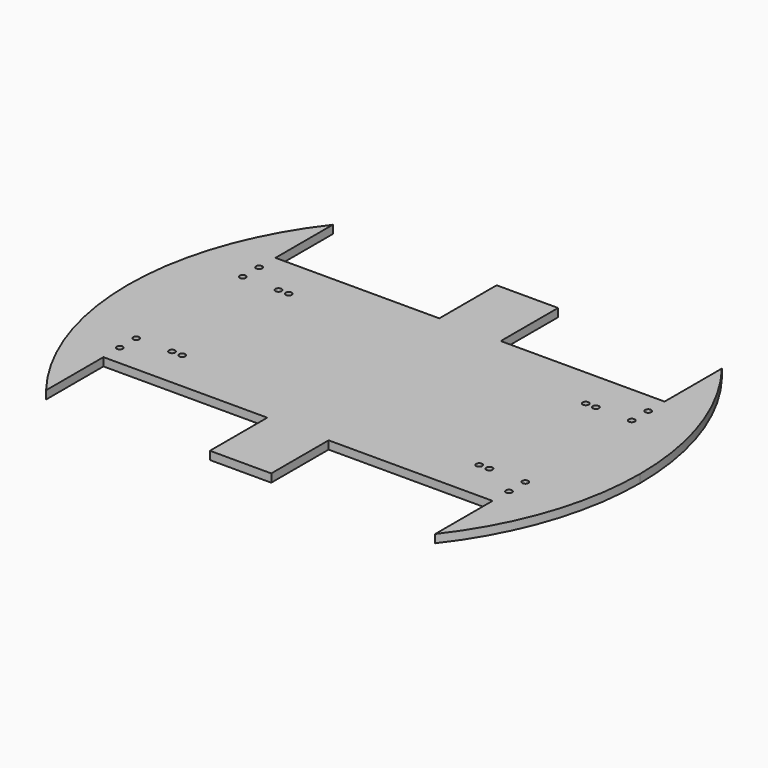
from build123d import *

# Parameters (mm, degrees)
F0_W     = 15
F0_H     = 4.4212083991
F0_H_2   = 48.0787916009
F0_W_2   = 29.9482679234
F0_H_3   = 35
F1_DEPTH = 4
F2_DEPTH = 4


with BuildPart() as f1:
    # F0 (on Top) → F1 (new body)
    with BuildSketch(Plane.XY):
        with BuildLine():
            Line((-125.2771986143, 41.785060304), (-125.2771986143, 50.285060304))
            Line((-125.2771986143, 50.285060304), (-125.2771986143, 85.285060304))
            ThreePointArc((-125.2771986143, 85.285060304), (-147.5688652809, 44.035060304), (-155.2771986143, -2.214939696))
            Line((-155.2771986143, -2.214939696), (-125.2771986143, -2.214939696))
            Line((-125.2771986143, -2.214939696), (-125.2771986143, 28.785060304))
            ThreePointArc((-125.2771986143, 28.785060304), (-126.7771986143, 30.285060304), (-125.2771986143, 31.785060304))
            Line((-125.2771986143, 31.785060304), (-125.2771986143, 38.785060304))
            ThreePointArc((-125.2771986143, 38.785060304), (-126.7771986143, 40.285060304), (-125.2771986143, 41.785060304))
        make_face()
        with BuildLine():
            Line((-85.2771986143, 50.285060304), (-125.2771986143, 50.285060304))
            Line((-125.2771986143, 50.285060304), (-125.2771986143, 41.785060304))
            ThreePointArc((-125.2771986143, 41.785060304), (-124.2165384425, 41.3457204758), (-123.7771986143, 40.285060304))
            ThreePointArc((-123.7771986143, 40.285060304), (-124.2165384425, 39.2244001322), (-125.2771986143, 38.785060304))
            Line((-125.2771986143, 38.785060304), (-125.2771986143, 31.785060304))
            ThreePointArc((-125.2771986143, 31.785060304), (-124.2165384425, 31.3457204758), (-123.7771986143, 30.285060304))
            ThreePointArc((-123.7771986143, 30.285060304), (-124.2165384425, 29.2244001322), (-125.2771986143, 28.785060304))
            Line((-125.2771986143, 28.785060304), (-125.2771986143, -2.214939696))
            Line((-125.2771986143, -2.214939696), (-107.7771986143, -2.214939696))
            Line((-107.7771986143, -2.214939696), (-102.7771986143, -2.214939696))
            Line((-102.7771986143, -2.214939696), (-85.2771986143, -2.214939696))
            Line((-85.2771986143, -2.214939696), (-85.2771986143, 50.285060304))
        make_face()
        with BuildLine():
            ThreePointArc((-106.2771986143, 30.285060304), (-106.7165384425, 29.2244001322), (-107.7771986143, 28.785060304))
            ThreePointArc((-107.7771986143, 28.785060304), (-108.837858786, 31.3457204758), (-106.2771986143, 30.285060304))
        make_face(mode=Mode.SUBTRACT)
        with BuildLine():
            ThreePointArc((-101.2771986143, 30.285060304), (-101.7165384425, 29.2244001322), (-102.7771986143, 28.785060304))
            ThreePointArc((-102.7771986143, 28.785060304), (-103.837858786, 31.3457204758), (-101.2771986143, 30.285060304))
        make_face(mode=Mode.SUBTRACT)
        Polygon((-45.2771986143, 50.285060304), (-85.2771986143, 50.285060304), (-85.2771986143, -2.214939696), (-45.2771986143, -2.214939696), (-45.2771986143, 45.8638519049), align=None)
        with Locations((-37.7771986143, 48.0744561044)):
            Rectangle(F0_W, F0_H)
        Polygon((-45.2771986143, 85.285060304), (-45.2771986143, 50.285060304), (-30.2771986143, 50.285060304), (-15.2771986143, 50.285060304), (-15.2771986143, 85.285060304), align=None)
        Polygon((-45.2771986143, -2.214939696), (-85.2771986143, -2.214939696), (-85.2771986143, -34.714939696), (-85.2771986143, -54.714939696), (-45.2771986143, -54.714939696), align=None)
        with BuildLine():
            Line((-125.2771986143, -2.214939696), (-155.2771986143, -2.214939696))
            ThreePointArc((-155.2771986143, -2.214939696), (-147.5688652809, -48.464939696), (-125.2771986143, -89.714939696))
            Line((-125.2771986143, -89.714939696), (-125.2771986143, -54.714939696))
            Line((-125.2771986143, -54.714939696), (-125.2771986143, -46.214939696))
            ThreePointArc((-125.2771986143, -46.214939696), (-126.7771986143, -44.714939696), (-125.2771986143, -43.214939696))
            Line((-125.2771986143, -43.214939696), (-125.2771986143, -36.214939696))
            ThreePointArc((-125.2771986143, -36.214939696), (-126.7771986143, -34.714939696), (-125.2771986143, -33.214939696))
            Line((-125.2771986143, -33.214939696), (-125.2771986143, -2.214939696))
        make_face()
        with Locations((-37.7771986143, 21.8244561044)):
            Rectangle(F0_W, F0_H_2)
        with Locations((-22.7771986143, 48.0744561044)):
            Rectangle(F0_W, F0_H)
        Polygon((-30.2771986143, -2.214939696), (-45.2771986143, -2.214939696), (-45.2771986143, -54.714939696), (-15.3289306909, -54.714939696), (-15.2771986143, -54.714939696), (-15.2771986143, -2.214939696), align=None)
        with Locations((-22.7771986143, 21.8244561044)):
            Rectangle(F0_W, F0_H_2)
        with BuildLine():
            Line((64.7228013857, 50.285060304), (-15.2771986143, 50.285060304))
            Line((-15.2771986143, 50.285060304), (-15.2771986143, 45.8638519049))
            Line((-15.2771986143, 45.8638519049), (-15.2771986143, -2.214939696))
            Line((-15.2771986143, -2.214939696), (42.2228013857, -2.214939696))
            Line((42.2228013857, -2.214939696), (42.2228013857, 28.785060304))
            ThreePointArc((42.2228013857, 28.785060304), (41.162141214, 31.3457204758), (43.7228013857, 30.285060304))
            Line((43.7228013857, 30.285060304), (45.7228013857, 30.285060304))
            ThreePointArc((45.7228013857, 30.285060304), (47.2228013857, 31.785060304), (48.7228013857, 30.285060304))
            Line((48.7228013857, 30.285060304), (63.2228013857, 30.285060304))
            ThreePointArc((63.2228013857, 30.285060304), (63.662141214, 31.3457204758), (64.7228013857, 31.785060304))
            Line((64.7228013857, 31.785060304), (64.7228013857, 38.785060304))
            ThreePointArc((64.7228013857, 38.785060304), (63.2228013857, 40.285060304), (64.7228013857, 41.785060304))
            Line((64.7228013857, 41.785060304), (64.7228013857, 50.285060304))
        make_face()
        with Locations((-30.3030646526, -72.214939696)):
            Rectangle(F0_W_2, F0_H_3)
        with BuildLine():
            Line((64.7228013857, 85.285060304), (64.7228013857, 50.285060304))
            Line((64.7228013857, 50.285060304), (64.7228013857, 41.785060304))
            ThreePointArc((64.7228013857, 41.785060304), (65.7834615575, 41.3457204758), (66.2228013857, 40.285060304))
            ThreePointArc((66.2228013857, 40.285060304), (65.7834615575, 39.2244001322), (64.7228013857, 38.785060304))
            Line((64.7228013857, 38.785060304), (64.7228013857, 31.785060304))
            ThreePointArc((64.7228013857, 31.785060304), (65.7834615575, 31.3457204758), (66.2228013857, 30.285060304))
            ThreePointArc((66.2228013857, 30.285060304), (65.7834615575, 29.2244001322), (64.7228013857, 28.785060304))
            Line((64.7228013857, 28.785060304), (64.7228013857, -2.214939696))
            Line((64.7228013857, -2.214939696), (94.7228013857, -2.214939696))
            ThreePointArc((94.7228013857, -2.214939696), (87.0144680524, 44.035060304), (64.7228013857, 85.285060304))
        make_face()
        with BuildLine():
            Line((42.2228013857, -2.214939696), (-15.2771986143, -2.214939696))
            Line((-15.2771986143, -2.214939696), (-15.2771986143, -54.714939696))
            Line((-15.2771986143, -54.714939696), (64.7228013857, -54.714939696))
            Line((64.7228013857, -54.714939696), (64.7228013857, -46.214939696))
            ThreePointArc((64.7228013857, -46.214939696), (63.2228013857, -44.714939696), (64.7228013857, -43.214939696))
            Line((64.7228013857, -43.214939696), (64.7228013857, -36.214939696))
            ThreePointArc((64.7228013857, -36.214939696), (63.2228013857, -34.714939696), (64.7228013857, -33.214939696))
            Line((64.7228013857, -33.214939696), (64.7228013857, -2.214939696))
            Line((64.7228013857, -2.214939696), (47.2228013857, -2.214939696))
            Line((47.2228013857, -2.214939696), (42.2228013857, -2.214939696))
        make_face()
        with BuildLine():
            ThreePointArc((43.7228013857, -34.714939696), (41.162141214, -35.7755998678), (42.2228013857, -33.214939696))
            ThreePointArc((42.2228013857, -33.214939696), (43.2834615575, -33.6542795242), (43.7228013857, -34.714939696))
        make_face(mode=Mode.SUBTRACT)
        with BuildLine():
            ThreePointArc((48.7228013857, -34.714939696), (46.162141214, -35.7755998678), (47.2228013857, -33.214939696))
            ThreePointArc((47.2228013857, -33.214939696), (48.2834615575, -33.6542795242), (48.7228013857, -34.714939696))
        make_face(mode=Mode.SUBTRACT)
        with BuildLine():
            Line((42.2228013857, 28.785060304), (42.2228013857, -2.214939696))
            Line((42.2228013857, -2.214939696), (47.2228013857, -2.214939696))
            Line((47.2228013857, -2.214939696), (47.2228013857, 28.785060304))
            ThreePointArc((47.2228013857, 28.785060304), (46.162141214, 29.2244001322), (45.7228013857, 30.285060304))
            Line((45.7228013857, 30.285060304), (43.7228013857, 30.285060304))
            ThreePointArc((43.7228013857, 30.285060304), (43.2834615575, 29.2244001322), (42.2228013857, 28.785060304))
        make_face()
        with BuildLine():
            ThreePointArc((64.7228013857, -89.714939696), (87.0144680524, -48.464939696), (94.7228013857, -2.214939696))
            Line((94.7228013857, -2.214939696), (64.7228013857, -2.214939696))
            Line((64.7228013857, -2.214939696), (64.7228013857, -33.214939696))
            ThreePointArc((64.7228013857, -33.214939696), (65.7834615575, -33.6542795242), (66.2228013857, -34.714939696))
            ThreePointArc((66.2228013857, -34.714939696), (65.7834615575, -35.7755998678), (64.7228013857, -36.214939696))
            Line((64.7228013857, -36.214939696), (64.7228013857, -43.214939696))
            ThreePointArc((64.7228013857, -43.214939696), (65.7834615575, -43.6542795242), (66.2228013857, -44.714939696))
            ThreePointArc((66.2228013857, -44.714939696), (65.7834615575, -45.7755998678), (64.7228013857, -46.214939696))
            Line((64.7228013857, -46.214939696), (64.7228013857, -54.714939696))
            Line((64.7228013857, -54.714939696), (64.7228013857, -89.714939696))
        make_face()
        with BuildLine():
            Line((47.2228013857, 28.785060304), (47.2228013857, -2.214939696))
            Line((47.2228013857, -2.214939696), (64.7228013857, -2.214939696))
            Line((64.7228013857, -2.214939696), (64.7228013857, 28.785060304))
            ThreePointArc((64.7228013857, 28.785060304), (63.662141214, 29.2244001322), (63.2228013857, 30.285060304))
            Line((63.2228013857, 30.285060304), (48.7228013857, 30.285060304))
            ThreePointArc((48.7228013857, 30.285060304), (48.2834615575, 29.2244001322), (47.2228013857, 28.785060304))
        make_face()
    extrude(amount=F1_DEPTH)

    # F0 (on Top) → F2 (join)
    with BuildSketch(Plane.XY):
        with BuildLine():
            Line((-85.2771986143, -54.714939696), (-85.2771986143, -34.714939696))
            Line((-85.2771986143, -34.714939696), (-101.2771986143, -34.714939696))
            ThreePointArc((-101.2771986143, -34.714939696), (-102.7771986143, -36.214939696), (-104.2771986143, -34.714939696))
            ThreePointArc((-104.2771986143, -34.714939696), (-105.2771986143, -35.714939696), (-106.2771986143, -34.714939696))
            ThreePointArc((-106.2771986143, -34.714939696), (-108.837858786, -35.7755998678), (-107.7771986143, -33.214939696))
            Line((-107.7771986143, -33.214939696), (-107.7771986143, -2.214939696))
            Line((-107.7771986143, -2.214939696), (-125.2771986143, -2.214939696))
            Line((-125.2771986143, -2.214939696), (-125.2771986143, -33.214939696))
            ThreePointArc((-125.2771986143, -33.214939696), (-124.2165384425, -33.6542795242), (-123.7771986143, -34.714939696))
            ThreePointArc((-123.7771986143, -34.714939696), (-124.2165384425, -35.7755998678), (-125.2771986143, -36.214939696))
            Line((-125.2771986143, -36.214939696), (-125.2771986143, -43.214939696))
            ThreePointArc((-125.2771986143, -43.214939696), (-124.2165384425, -43.6542795242), (-123.7771986143, -44.714939696))
            ThreePointArc((-123.7771986143, -44.714939696), (-124.2165384425, -45.7755998678), (-125.2771986143, -46.214939696))
            Line((-125.2771986143, -46.214939696), (-125.2771986143, -54.714939696))
            Line((-125.2771986143, -54.714939696), (-85.2771986143, -54.714939696))
        make_face()
        with BuildLine():
            ThreePointArc((-106.2771986143, -34.714939696), (-105.2771986143, -35.714939696), (-104.2771986143, -34.714939696))
            Line((-104.2771986143, -34.714939696), (-105.2771986143, -34.714939696))
            Line((-105.2771986143, -34.714939696), (-106.2771986143, -34.714939696))
        make_face()
        with BuildLine():
            Line((-105.2771986143, -34.714939696), (-104.2771986143, -34.714939696))
            ThreePointArc((-104.2771986143, -34.714939696), (-105.2771986143, -33.714939696), (-106.2771986143, -34.714939696))
            Line((-106.2771986143, -34.714939696), (-105.2771986143, -34.714939696))
        make_face()
        with BuildLine():
            Line((-102.7771986143, -33.214939696), (-102.7771986143, -2.214939696))
            Line((-102.7771986143, -2.214939696), (-107.7771986143, -2.214939696))
            Line((-107.7771986143, -2.214939696), (-107.7771986143, -33.214939696))
            ThreePointArc((-107.7771986143, -33.214939696), (-106.7165384425, -33.6542795242), (-106.2771986143, -34.714939696))
            ThreePointArc((-106.2771986143, -34.714939696), (-105.2771986143, -33.714939696), (-104.2771986143, -34.714939696))
            ThreePointArc((-104.2771986143, -34.714939696), (-103.837858786, -33.6542795242), (-102.7771986143, -33.214939696))
        make_face()
        with BuildLine():
            Line((-85.2771986143, -34.714939696), (-85.2771986143, -2.214939696))
            Line((-85.2771986143, -2.214939696), (-102.7771986143, -2.214939696))
            Line((-102.7771986143, -2.214939696), (-102.7771986143, -33.214939696))
            ThreePointArc((-102.7771986143, -33.214939696), (-101.7165384425, -33.6542795242), (-101.2771986143, -34.714939696))
            Line((-101.2771986143, -34.714939696), (-85.2771986143, -34.714939696))
        make_face()
        with BuildLine():
            Line((42.2228013857, -2.214939696), (-15.2771986143, -2.214939696))
            Line((-15.2771986143, -2.214939696), (-15.2771986143, -54.714939696))
            Line((-15.2771986143, -54.714939696), (64.7228013857, -54.714939696))
            Line((64.7228013857, -54.714939696), (64.7228013857, -46.214939696))
            ThreePointArc((64.7228013857, -46.214939696), (63.2228013857, -44.714939696), (64.7228013857, -43.214939696))
            Line((64.7228013857, -43.214939696), (64.7228013857, -36.214939696))
            ThreePointArc((64.7228013857, -36.214939696), (63.2228013857, -34.714939696), (64.7228013857, -33.214939696))
            Line((64.7228013857, -33.214939696), (64.7228013857, -2.214939696))
            Line((64.7228013857, -2.214939696), (47.2228013857, -2.214939696))
            Line((47.2228013857, -2.214939696), (42.2228013857, -2.214939696))
        make_face()
        with BuildLine():
            ThreePointArc((43.7228013857, -34.714939696), (41.162141214, -35.7755998678), (42.2228013857, -33.214939696))
            ThreePointArc((42.2228013857, -33.214939696), (43.2834615575, -33.6542795242), (43.7228013857, -34.714939696))
        make_face(mode=Mode.SUBTRACT)
        with BuildLine():
            ThreePointArc((48.7228013857, -34.714939696), (46.162141214, -35.7755998678), (47.2228013857, -33.214939696))
            ThreePointArc((47.2228013857, -33.214939696), (48.2834615575, -33.6542795242), (48.7228013857, -34.714939696))
        make_face(mode=Mode.SUBTRACT)
    extrude(amount=F2_DEPTH)


solid = f1.part
